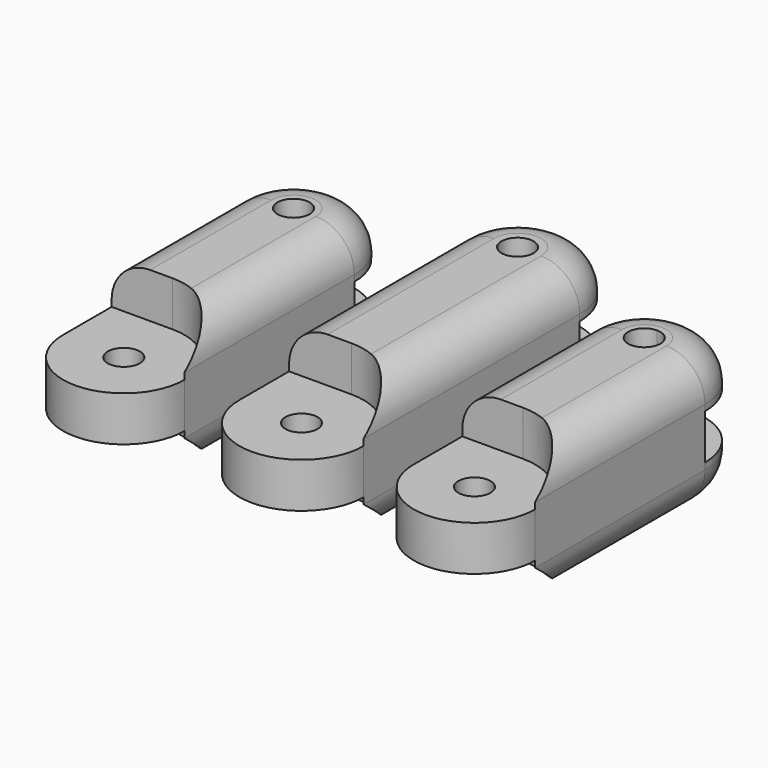
from build123d import *

# Parameters (mm, degrees)
F1_DEPTH   = 8.89
F3_DEPTH   = 8.89
F5_DEPTH   = 8.89
F6_D       = 6.35
F6_DEPTH   = 17.781
F6_ON_F0_D = 6.35
F7_D       = 6.35
F8_R       = 7.62
F10_DEPTH  = 8.89
F12_DEPTH  = 8.89
F14_DEPTH  = 8.89
F15_D      = 6.35
F16_D      = 6.35
F17_R      = 7.62
F19_DEPTH  = 8.89
F21_DEPTH  = 8.89
F23_DEPTH  = 8.89
F24_D      = 6.35
F25_D      = 6.35
F25_DEPTH  = 8.891
F26_R      = 7.62
F27_D      = 6.35


with BuildPart() as f1:
    # F0 (on Top) → F1 (new body)
    with BuildSketch(Plane.XY):
        with BuildLine():
            ThreePointArc((-59.256437, 12.0015), (-50.770095, 8.486342), (-47.254937, 0))
            Line((-47.254937, 0), (-47.254937, 41.91))
            ThreePointArc((-47.254937, 41.91), (-59.256437, 53.9115), (-71.257937, 41.91))
            Line((-71.257937, 41.91), (-71.257937, 12.0015))
            Line((-71.257937, 12.0015), (-59.256437, 12.0015))
        make_face()
    extrude(amount=F1_DEPTH)

    # F2 (on face) → F3 (join)
    with BuildSketch(Plane.XY.offset(8.89)):
        with BuildLine():
            ThreePointArc((-47.254937, 41.91), (-50.770095, 33.423658), (-59.256437, 29.9085))
            Line((-59.256437, 29.9085), (-71.257937, 29.9085))
            Line((-71.257937, 29.9085), (-71.257937, 0))
            ThreePointArc((-71.257937, 0), (-59.256437, -12.0015), (-47.254937, 0))
            Line((-47.254937, 0), (-47.254937, 41.91))
        make_face()
    extrude(amount=F3_DEPTH)

    # F4 (on face) → F5 (join)
    with BuildSketch(Plane.XY.offset(17.78)):
        with BuildLine():
            ThreePointArc((-59.256437, 12.0015), (-50.770095, 8.486342), (-47.254937, 0))
            Line((-47.254937, 0), (-47.254937, 41.91))
            ThreePointArc((-47.254937, 41.91), (-59.244549, 53.911506), (-71.257937, 41.933801))
            Line((-71.257937, 41.933801), (-71.257937, 12.0015))
            Line((-71.257937, 12.0015), (-59.256437, 12.0015))
        make_face()
    extrude(amount=F5_DEPTH)

    # F6 (through all, one way)
    with BuildSketch(Plane(origin=(0, 0, 8.89), x_dir=(1, 0, 0), z_dir=(0, 0, -1))):
        with Locations((-59.256437, -41.91)):
            Circle(F6_D / 2)
    extrude(amount=-F6_DEPTH, mode=Mode.SUBTRACT)

    # F6 on F0 (through all)
    with Locations(Plane(origin=(0, 0, 0), x_dir=(1, 0, 0), z_dir=(0, 0, -1))):
        with Locations((-59.256437, -41.91)):
            Hole(F6_ON_F0_D / 2)

    # F7 (through all)
    with Locations(Plane(origin=(0, 0, 8.89), x_dir=(1, 0, 0), z_dir=(0, 0, -1))):
        with Locations((-59.256437, 0)):
            Hole(F7_D / 2)

    # F8
    f8_edges = [f1.edges().sort_by_distance(p)[0] for p in [
        (-47.254937, 20.955, 26.67),
        (-71.257937, 26.967651, 26.67),
        (-47.254937, 20.955, 0),
    ]]
    fillet(f8_edges, radius=F8_R)


with BuildPart() as f10:
    # F9 (on Top) → F10 (new body)
    with BuildSketch(Plane.XY):
        with BuildLine():
            ThreePointArc((-24.152765, 12.279155), (-15.470091, 8.682674), (-11.87361, 0))
            Line((-11.87361, 0), (-11.87361, 53.34))
            ThreePointArc((-11.87361, 53.34), (-24.152765, 65.619155), (-36.43192, 53.34))
            Line((-36.43192, 53.34), (-36.43192, 12.279155))
            Line((-36.43192, 12.279155), (-24.152765, 12.279155))
        make_face()
    extrude(amount=F10_DEPTH)

    # F11 (on face) → F12 (join)
    with BuildSketch(Plane.XY.offset(8.89)):
        with BuildLine():
            ThreePointArc((-11.87361, 53.34), (-15.470091, 44.657326), (-24.152765, 41.060845))
            Line((-24.152765, 41.060845), (-36.43192, 41.060845))
            Line((-36.43192, 41.060845), (-36.43192, 0))
            ThreePointArc((-36.43192, 0), (-24.152765, -12.279155), (-11.87361, 0))
            Line((-11.87361, 0), (-11.87361, 53.34))
        make_face()
    extrude(amount=F12_DEPTH)

    # F13 (on face) → F14 (join)
    with BuildSketch(Plane.XY.offset(17.78)):
        with BuildLine():
            Line((-11.87361, 0), (-11.87361, 53.34))
            ThreePointArc((-11.87361, 53.34), (-24.152901, 65.619019), (-36.431648, 53.339455))
            Line((-36.431648, 53.339455), (-36.431858, 12.279155))
            Line((-36.431858, 12.279155), (-24.152765, 12.279155))
            ThreePointArc((-24.152765, 12.279155), (-15.470091, 8.682674), (-11.87361, 0))
        make_face()
    extrude(amount=F14_DEPTH)

    # F15 (through all)
    with Locations(Plane(origin=(0, 0, 8.89), x_dir=(1, 0, 0), z_dir=(0, 0, -1))):
        with Locations((-24.152765, 0)):
            Hole(F15_D / 2)

    # F16 (through all)
    with Locations(Plane(origin=(0, 0, 0), x_dir=(1, 0, 0), z_dir=(0, 0, -1))):
        with Locations((-24.152765, -53.34)):
            Hole(F16_D / 2)

    # F17
    f17_edges = [f10.edges().sort_by_distance(p)[0] for p in [
        (-36.43192, 32.809578, 0),
        (-11.87361, 26.67, 26.67),
    ]]
    fillet(f17_edges, radius=F17_R)


with BuildPart() as f19:
    # F18 (on Top) → F19 (new body)
    with BuildSketch(Plane.XY):
        with BuildLine():
            ThreePointArc((10.006107, 12.0015), (18.492449, 8.486342), (22.007607, 0))
            Line((22.007607, 0), (22.007607, 41.91))
            ThreePointArc((22.007607, 41.91), (10.006107, 53.9115), (-1.995393, 41.91))
            Line((-1.995393, 41.91), (-1.995393, 12.0015))
            Line((-1.995393, 12.0015), (10.006107, 12.0015))
        make_face()
    extrude(amount=F19_DEPTH)

    # F20 (on face) → F21 (join)
    with BuildSketch(Plane.XY.offset(8.89)):
        with BuildLine():
            Line((22.007607, 0), (22.007607, 41.91))
            ThreePointArc((22.007607, 41.91), (18.492449, 33.423658), (10.006107, 29.9085))
            Line((10.006107, 29.9085), (-1.995393, 29.9085))
            Line((-1.995393, 29.9085), (-1.995393, 0))
            ThreePointArc((-1.995393, 0), (10.006107, -12.0015), (22.007607, 0))
        make_face()
    extrude(amount=F21_DEPTH)

    # F22 (on face) → F23 (join)
    with BuildSketch(Plane.XY.offset(17.78)):
        with BuildLine():
            Line((22.007607, 0), (22.007607, 41.91))
            ThreePointArc((22.007607, 41.91), (10.00515, 53.910922), (-1.994237, 41.906931))
            Line((-1.994237, 41.906931), (-1.995062, 12.0015))
            Line((-1.995062, 12.0015), (10.006107, 12.0015))
            ThreePointArc((10.006107, 12.0015), (18.492449, 8.486342), (22.007607, 0))
        make_face()
    extrude(amount=F23_DEPTH)

    # F24 (through all)
    with Locations(Plane.XY.offset(17.78)):
        with Locations((10.006107, 0)):
            Hole(F24_D / 2)

    # F25 (through all, one way)
    with BuildSketch(Plane(origin=(0, 0, 17.78), x_dir=(1, 0, 0), z_dir=(0, 0, -1))):
        with Locations((10.006685, -41.91)):
            Circle(F25_D / 2)
    extrude(amount=-F25_DEPTH, mode=Mode.SUBTRACT)

    # F26
    f26_edges = [f19.edges().sort_by_distance(p)[0] for p in [
        (22.007607, 20.955, 26.67),
        (22.007607, 20.955, 0),
    ]]
    fillet(f26_edges, radius=F26_R)

    # F27 (through all)
    with Locations(Plane(origin=(0, 0, 0), x_dir=(1, 0, 0), z_dir=(0, 0, -1))):
        with Locations((10.006107, -41.91)):
            Hole(F27_D / 2)


solid = Compound([f1.part, f10.part, f19.part])
